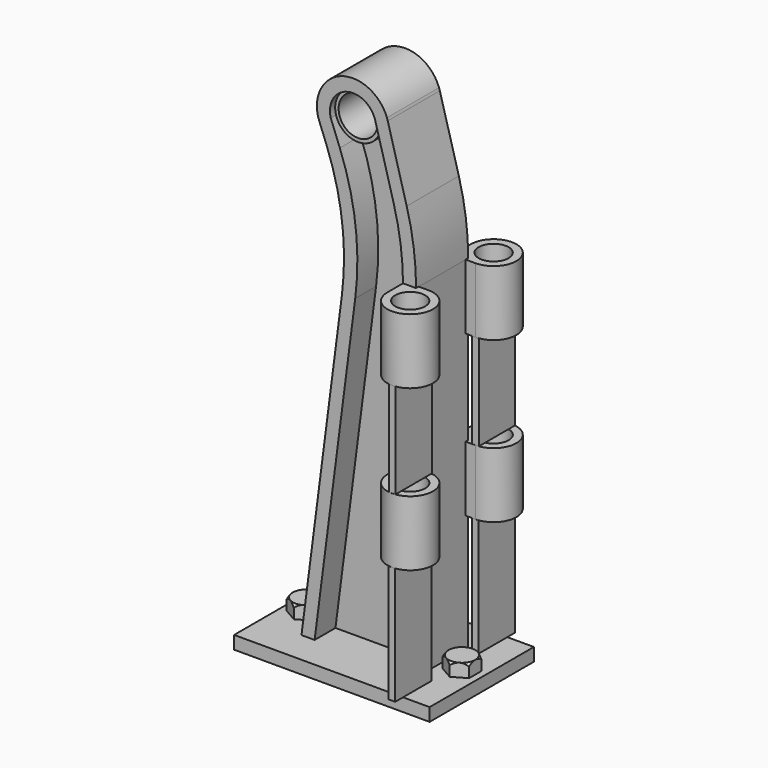
from build123d import *

# Parameters (mm, degrees)
F1_DEPTH    = 2.5
F2_R        = 20
F3_T1_DEPTH = 7.2919338558
F3_T3_DEPTH = 5.7629746737
F5_DEPTH    = 2
F6_R        = 20
F8_DEPTH    = 2
F9_W        = 15
F9_H        = 10
F10_DEPTH   = 1
F12_R       = 20
F13_R       = 1.15
F14_DEPTH   = 17.3
F16_W       = 4
F16_H       = 7.3
F17_DEPTH   = 25
F19_D       = 3
F19_DEPTH   = 5
F19_TIP     = 0.9012909285
F20_R       = 1.7700631876
F20_R_2     = 1.5
F21_DEPTH   = 2
F22_W       = 4
F22_H       = 7.3
F23_DEPTH   = 12.5
F24_DEPTH   = 2
F26_DEPTH   = 1
F30_W       = 0.5
F30_H       = 3.5
F31_DEPTH   = 9
F32_W       = 0.5
F32_H       = 3.5
F33_DEPTH   = 7.3


# Not quite as in the source:
# - a fillet or chamfer that OpenCascade refuses, or shapes differently, is made with other operations: its cross-section is extruded or revolved along the edge and cut away or added
# - ends of sketch curves that miss each other by under 0.0002 mm in the source are joined
# - a feature names something its author has since deleted; it is built from what else it names


with BuildPart() as f1:
    # F0 (on Front) → F1 (new body, symmetric)
    with BuildSketch(Plane.XZ):
        with BuildLine():
            Line((-4.461364258, 0), (4.4613697168, 0))
            Line((4.4613697168, 0), (4.4613697168, 30))
            Line((4.4613697168, 30), (2.2730625034, 37.9387021101))
            ThreePointArc((2.2730625034, 37.9387021101), (-1.1809999696, 39.7873473063), (-3.0296451657, 36.3332848334))
            Line((-3.0296451657, 36.3332848334), (-0.5806429216, 30.0000008653))
            Line((-0.5806429216, 30.0000008653), (-4.461364258, 0))
        make_face()
    extrude(amount=F1_DEPTH, both=True)

    # F2
    f2_edges = [f1.edges().sort_by_distance(p)[0] for p in [
        (4.46137, 0, 30),
        (-0.580643, 0, 30.000001),
    ]]
    fillet(f2_edges, radius=F2_R)

    # F3: fillet of radius 2.5 on 3 edges, made by hand

    # F3_s2 → F3_t1 (cut)
    with BuildSketch(Plane.XZ.offset(-3.6459669279)):
        with BuildLine():
            ThreePointArc((-3.1257167168, 36.7814909121), (-3.0693855707, 36.4861770404), (-2.9780129086, 36.1997603554))
            Line((-2.9780129086, 36.1997603554), (-3.0296451657, 36.3332848334))
            ThreePointArc((-3.0296451657, 36.3332848334), (-3.0869674726, 36.5553973342), (-3.1257167168, 36.7814909121))
        make_face()
    extrude(amount=F3_T1_DEPTH, mode=Mode.SUBTRACT)

    # F3_s4 → F3_t3 (cut)
    with BuildSketch(Plane.XZ.offset(-2.8814873369)):
        with BuildLine():
            ThreePointArc((2.2857269032, 37.8927584249), (2.257193358, 37.9887275108), (2.2248400544, 38.0834771409))
            ThreePointArc((2.2248400544, 38.0834771409), (2.2499483239, 38.0114217266), (2.2730625034, 37.9387021101))
            Line((2.2730625034, 37.9387021101), (2.2857269032, 37.8927584249))
        make_face()
    extrude(amount=F3_T3_DEPTH, mode=Mode.SUBTRACT)

    # F4 (on face) → F5 (cut)
    with BuildSketch(Plane.XZ.offset(2.5)):
        with BuildLine():
            Line((-3.3236755119, 0.999999488), (3.4613702287, 0.999999488))
            Line((3.4613702287, 0.999999488), (3.4613702287, 29.8646979397))
            Line((3.4613702287, 29.8646979397), (1.3127120624, 37.6595619399))
            ThreePointArc((1.3127120624, 37.6595619399), (-0.880587822, 38.8334370358), (-2.0819074864, 36.6550481386))
            Line((-2.0819074864, 36.6550481386), (0.4436883577, 30.1236879865))
            Line((0.4436883577, 30.1236879865), (-3.3236755119, 0.999999488))
        make_face()
    extrude(amount=-F5_DEPTH, mode=Mode.SUBTRACT)

    # F6
    f6_edges = [f1.edges().sort_by_distance(p)[0] for p in [
        (0.443688, -1.5, 30.123688),
        (3.46137, -1.5, 29.864698),
    ]]
    fillet(f6_edges, radius=F6_R)

    # F7 (on face) → F8 (cut)
    with BuildSketch(Plane(origin=(0, 2.5, 0), x_dir=(-1, 0, 0), z_dir=(0, 1, 0))):
        with BuildLine():
            Line((-3.4613697168, 29.8646984516), (-3.4613697168, 1))
            Line((-3.4613697168, 1), (3.3236760239, 1))
            Line((3.3236760239, 1), (-0.4436878458, 30.1236884984))
            Line((-0.4436878458, 30.1236884984), (2.0819079984, 36.6550486506))
            ThreePointArc((2.0819079984, 36.6550486506), (0.8805883339, 38.8334375478), (-1.3127115504, 37.6595624519))
            Line((-1.3127115504, 37.6595624519), (-3.4613697168, 29.8646984516))
        make_face()
    extrude(amount=-F8_DEPTH, mode=Mode.SUBTRACT)

    # F9 (on Top) → F10 (join)
    with BuildSketch(Plane.XY):
        Rectangle(F9_W, F9_H)
    extrude(amount=F10_DEPTH)

    # F12
    f12_edges = [f1.edges().sort_by_distance(p)[0] for p in [
        (0.443688, 1.5, 30.123688),
        (3.46137, 1.5, 29.864698),
    ]]
    fillet(f12_edges, radius=F12_R)

    # F13 (on offset) → F14 (join)
    with BuildSketch(Plane.XY.offset(10)):
        with BuildLine():
            ThreePointArc((3.4613697168, -4), (6.4488065838, -5.2374368671), (5.2113697168, -2.25))
            Line((5.2113697168, -2.25), (3.4613697168, -2.25))
            Line((3.4613697168, -2.25), (3.4613697168, -4))
        make_face()
        with Locations((5.2113697168, -4.00000019)):
            Circle(F13_R, mode=Mode.SUBTRACT)
        with BuildLine():
            Line((3.4613697168, 2.25), (5.2113697168, 2.25))
            ThreePointArc((5.2113697168, 2.25), (6.4488065838, 5.2374368671), (3.4613697168, 4))
            Line((3.4613697168, 4), (3.4613697168, 2.25))
        make_face()
        with Locations((5.2113697168, 4.00000019)):
            Circle(F13_R, mode=Mode.SUBTRACT)
    extrude(amount=F14_DEPTH)

    # F16 (on offset) → F17 (cut)
    with BuildSketch(Plane.YZ.offset(8)):
        with Locations((-4.5, 18.65)):
            Rectangle(F16_W, F16_H)
        with Locations((4.5, 18.65)):
            Rectangle(F16_W, F16_H)
    extrude(amount=-F17_DEPTH, mode=Mode.SUBTRACT)

    # F19
    with Locations(Plane(origin=(0, 0.5, 0), x_dir=(-1, 0, 0), z_dir=(0, 1, 0))):
        with Locations((0.384598224, 37.1573055512)):
            Hole(F19_D / 2, depth=F19_DEPTH)
            with Locations((0, 0, -(F19_DEPTH + F19_TIP / 2))):  # 118° drill point
                Cone(0, F19_D / 2, F19_TIP, mode=Mode.SUBTRACT)

    # F20 (on Front) → F21 (join)
    with BuildSketch(Plane.XZ):
        with Locations((-0.384598224, 37.1573055512)):
            Circle(F20_R)
        with Locations((-0.384598224, 37.1573055512)):
            Circle(F20_R_2, mode=Mode.SUBTRACT)
    extrude(amount=F21_DEPTH)

    # F22 (on Front) → F23 (cut, symmetric)
    with BuildSketch(Plane.XZ):
        with Locations((6.4613697168, 18.65)):
            Rectangle(F22_W, F22_H)
    extrude(amount=F23_DEPTH, both=True, mode=Mode.SUBTRACT)

    # F20 (on Front) → F24 (join)
    with BuildSketch(Plane.XZ):
        with Locations((-0.384598224, 37.1573055512)):
            Circle(F20_R)
        with Locations((-0.384598224, 37.1573055512)):
            Circle(F20_R_2, mode=Mode.SUBTRACT)
    extrude(amount=-F24_DEPTH)

    # F25 (on face) → F26 (join)
    with BuildSketch(Plane.XY.offset(0.999999488)):
        Polygon((7.001387421, -0.5893031513), (7.001387421, 0.5893031513), (5.980684422, 1.1786063026), (4.9599814229, 0.5893031513), (4.9599814229, -0.5893031513), (5.980684422, -1.1786063026), align=None)
        Polygon((-5.980684422, -1.1786063026), (-4.9599814229, -0.5893031513), (-4.9599814229, 0.5893031513), (-5.980684422, 1.1786063026), (-7.001387421, 0.5893031513), (-7.001387421, -0.5893031513), align=None)
    extrude(amount=F26_DEPTH)

    # F27 (on Front) → F28 (revolve, cut)
    with BuildSketch(Plane.XZ):
        Polygon((7.3244427331, 1.999999488), (7.001387421, 1.999999488), (7.3244427331, 1.5525314957), align=None)
    revolve(axis=Axis((5.980684422, 0, 1.2804081198), (0, 0, 1)), mode=Mode.SUBTRACT)

    # F27 (on Front) → F29 (revolve, cut)
    with BuildSketch(Plane.XZ):
        Polygon((-7.3244427331, 1.999999488), (-7.3244427331, 1.5525314957), (-7.001387421, 1.999999488), align=None)
    revolve(axis=Axis((-5.980684422, 0, 1.2804081198), (0, 0, 1)), mode=Mode.SUBTRACT)


with BuildPart() as f31:
    # F30 (on offset) → F31 (new body, through all)
    with BuildSketch(Plane.XY.offset(10)):
        with Locations((5.2113697168, 4)):
            Rectangle(F30_W, F30_H)
    extrude(amount=-F31_DEPTH)


with BuildPart() as f31b:
    # F30 (on offset) → F31, piece 2 (new body, through all)
    with BuildSketch(Plane.XY.offset(10)):
        with Locations((5.2113697168, -4)):
            Rectangle(F30_W, F30_H)
    extrude(amount=-F31_DEPTH)


with BuildPart() as f33:
    # F32 (on face) → F33 (new body, through all)
    with BuildSketch(Plane.XY.offset(15)):
        with Locations((5.2113697168, 4.0124509092)):
            Rectangle(F32_W, F32_H)
    extrude(amount=F33_DEPTH)


with BuildPart() as f33b:
    # F32 (on face) → F33, piece 2 (new body, through all)
    with BuildSketch(Plane.XY.offset(15)):
        Polygon((5.4613697168, -4.2375490908), (5.4613697168, -2.2375490908), (4.9613697168, -2.2375490908), (4.9613697168, -4.2375490908), (4.9613697168, -5.7375490908), (5.4613697168, -5.7375490908), align=None)
    extrude(amount=F33_DEPTH)


solid = Compound([f1.part, f31.part, f31b.part, f33.part, f33b.part])
